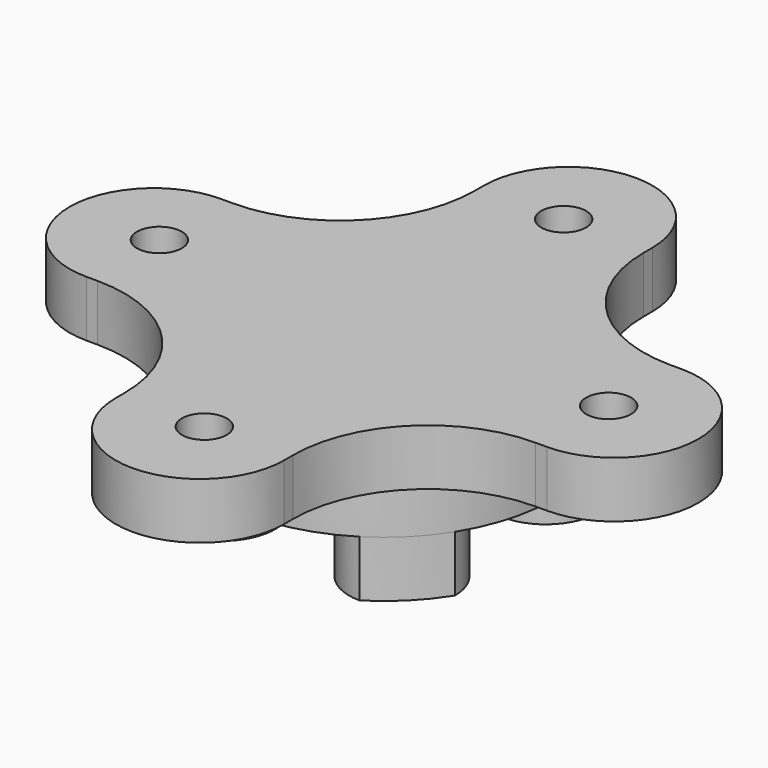
from build123d import *

# Parameters (mm, degrees)
F0_R     = 2
F1_DEPTH = 5
F2_R     = 15
F3_DEPTH = 4
F5_DEPTH = 5


# Not quite as in the source:
# - after a boolean that leaves OpenCascade's solid faulty, fix() repairs it


with BuildPart() as f1:
    # F0 (on Top) → F1 (new body)
    with BuildSketch(Plane.XY):
        with BuildLine():
            ThreePointArc((0, 28), (-5.3033008589, 25.8033008589), (-7.5, 20.5))
            Line((-7.5, 20.5), (-7.5, 19.5))
            ThreePointArc((-7.5, 19.5), (-11.0147186258, 11.0147186258), (-19.5, 7.5))
            Line((-19.5, 7.5), (-20.5, 7.5))
            ThreePointArc((-20.5, 7.5), (-25.8033008589, 5.3033008589), (-28, 0))
            ThreePointArc((-28, 0), (-25.8033008589, -5.3033008589), (-20.5, -7.5))
            Line((-20.5, -7.5), (-19.5, -7.5))
            ThreePointArc((-19.5, -7.5), (-11.0147186258, -11.0147186258), (-7.5, -19.5))
            Line((-7.5, -19.5), (-7.5, -20.5))
            ThreePointArc((-7.5, -20.5), (-5.3033008589, -25.8033008589), (0, -28))
            ThreePointArc((0, -28), (5.3033008589, -25.8033008589), (7.5, -20.5))
            Line((7.5, -20.5), (7.5, -19.5))
            ThreePointArc((7.5, -19.5), (11.0147186258, -11.0147186258), (19.5, -7.5))
            Line((19.5, -7.5), (20.5, -7.5))
            ThreePointArc((20.5, -7.5), (25.8033008589, -5.3033008589), (28, 0))
            ThreePointArc((28, 0), (25.8033008589, 5.3033008589), (20.5, 7.5))
            Line((20.5, 7.5), (19.5, 7.5))
            ThreePointArc((19.5, 7.5), (11.0147186258, 11.0147186258), (7.5, 19.5))
            Line((7.5, 19.5), (7.5, 20.5))
            ThreePointArc((7.5, 20.5), (5.3033008589, 25.8033008589), (0, 28))
        make_face()
        with Locations((0, -20)):
            Circle(F0_R, mode=Mode.SUBTRACT)
        with Locations((-20, 0)):
            Circle(F0_R, mode=Mode.SUBTRACT)
        with Locations((20, 0)):
            Circle(F0_R, mode=Mode.SUBTRACT)
        with Locations((0, 20)):
            Circle(F0_R, mode=Mode.SUBTRACT)
    extrude(amount=F1_DEPTH)

    # F2 (on Top) → F3 (join)
    with BuildSketch(Plane.XY):
        Circle(F2_R)
    extrude(amount=-F3_DEPTH)

    # F4 (on face) → F5 (join)
    with BuildSketch(Plane(origin=(0, 0, -4), x_dir=(1, 0, 0), z_dir=(0, 0, -1))):
        with BuildLine():
            ThreePointArc((-7.9819098145, 12.6999651855), (-10.6066017178, 10.6066017178), (-12.6999651855, 7.9819098145))
            ThreePointArc((-12.6999651855, 7.9819098145), (-4.6765981284, 4.6765981284), (-7.9819098145, 12.6999651855))
        make_face()
        with BuildLine():
            ThreePointArc((12.6999651855, 7.9819098145), (10.6066017178, 10.6066017178), (7.9819098145, 12.6999651855))
            ThreePointArc((7.9819098145, 12.6999651855), (4.6765981284, 4.6765981284), (12.6999651855, 7.9819098145))
        make_face()
        with BuildLine():
            ThreePointArc((7.9819098145, -12.6999651855), (10.6066017178, -10.6066017178), (12.6999651855, -7.9819098145))
            ThreePointArc((12.6999651855, -7.9819098145), (4.6765981284, -4.6765981284), (7.9819098145, -12.6999651855))
        make_face()
        with BuildLine():
            ThreePointArc((-12.6999651855, -7.9819098145), (-10.6066017178, -10.6066017178), (-7.9819098145, -12.6999651855))
            ThreePointArc((-7.9819098145, -12.6999651855), (-4.6765981284, -4.6765981284), (-12.6999651855, -7.9819098145))
        make_face()
    extrude(amount=F5_DEPTH)

    add(f1.part.fix(), mode=Mode.REPLACE)


solid = f1.part
